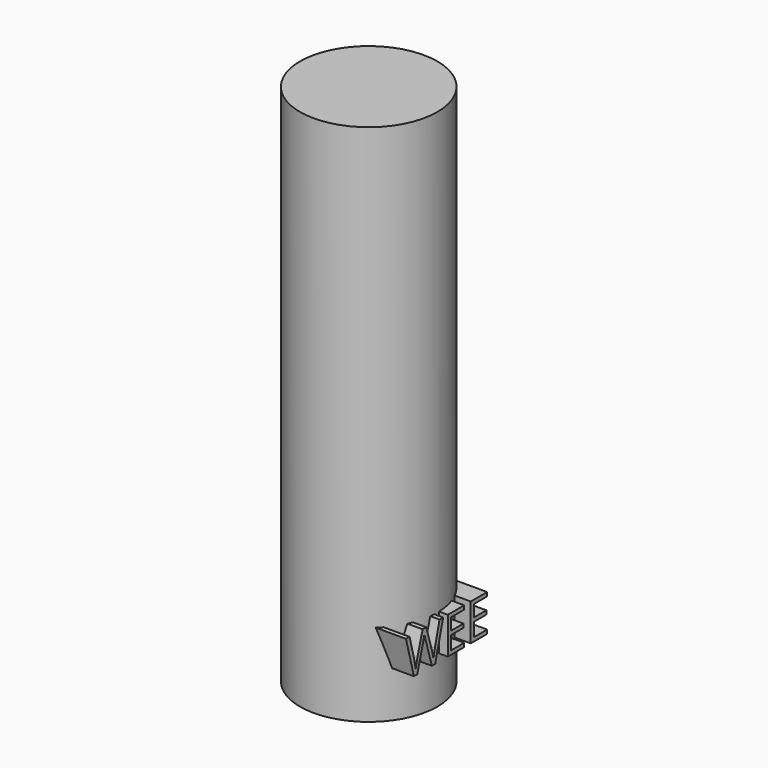
from build123d import *

# Parameters (mm, degrees)
F0_R         = 23.4398317113
F1_DEPTH     = 178.816
F2_TEXT_SIZE = 17.6388888889
F3_DEPTH     = 26.416


# Not quite as in the source:
# - Text() gives the source's letters only with a copy of the font that has no kerning and outlines rounded to 1/6400 em; it was checked with that copy


with BuildPart() as f1:
    # F0 (on Top) → F1 (new body)
    with BuildSketch(Plane.XY):
        Circle(F0_R)
    extrude(amount=F1_DEPTH)

    # F2 (on Right) → F3 (join)
    with BuildSketch(Plane.YZ):
        with Locations((-17.3237905203, 15.7177011008)):
            Text('WEE', F2_TEXT_SIZE, font='Open Sans', text_align=(TextAlign.LEFT, TextAlign.BOTTOM))
    extrude(amount=F3_DEPTH)


solid = f1.part
